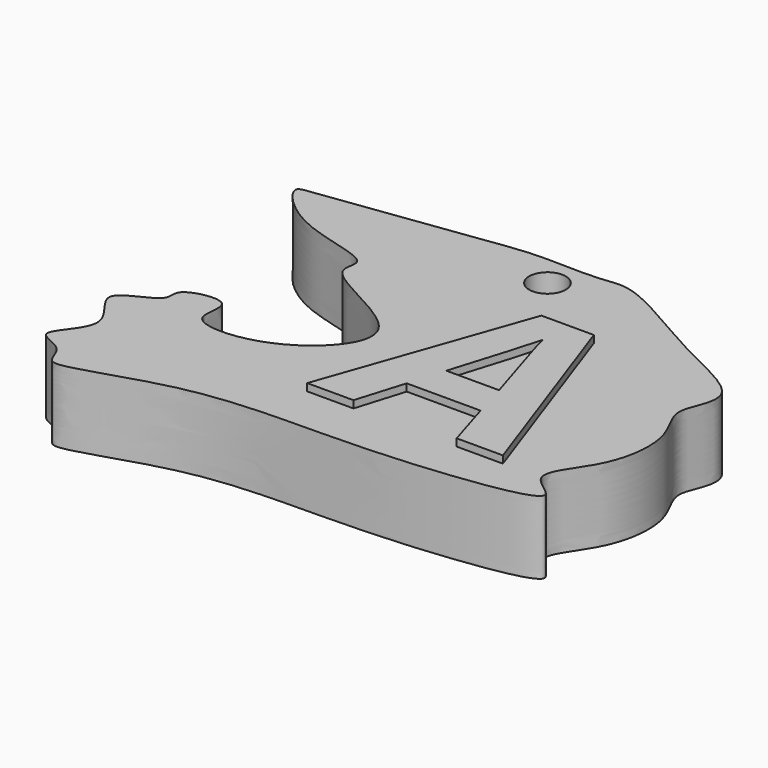
from build123d import *

# Parameters (mm, degrees)
F1_DEPTH     = 10
F2_TEXT_SIZE = 38.8719503664
F3_DEPTH     = 1
F5_D         = 5


# Not quite as in the source:
# - Text() gives the source's letters only with a copy of the font that has no kerning and outlines rounded to 1/6400 em; it was checked with that copy


with BuildPart() as f1:
    # F0 (on Top) → F1 (new body)
    with BuildSketch(Plane.XY):
        with BuildLine():
            add(Edge.make_bspline(
                [(-64.71713292, 51.556880079), (-62.588218655, 51.8064642414), (-54.5923947778, 52.9452082504), (-42.8082906348, 54.4694674172), (-36.54422944, 55.4457616296), (-28.0628023597, 54.8604905032), (-23.6071907873, 56.2361288313), (-11.7612832999, 48.5936441209), (-4.1799815494, 45.3962070939), (-0.4613117813, 42.5097622921), (-1.064368556, 39.231742487), (-2.8508041663, 35.8033968438), (1.0588645249, 31.1016218737), (0.1291140085, 21.6916004401), (-6.4423138044, 15.2417197866), (2.3773918907, 11.6389914958), (-14.074909308, 9.0603488589), (-29.0219761766, 8.4696762862), (-46.0852185761, 8.6454293617), (-59.7566922689, 3.1529002931), (-62.3297147196, 3.588226522), (-62.7184982721, 6.9655340487), (-68.4749409776, 7.8555551624), (-60.7053390885, 13.7573924), (-69.434806753, 19.8215393445), (-60.3239056166, 21.911121728), (-62.2881701416, 25.2528184799), (-54.4025753252, 26.8842302627), (-56.4195942983, 21.6120322246), (-53.1570896421, 19.8158876953), (-43.8341594361, 21.0472296338), (-33.803067045, 32.4464067053), (-52.7781031406, 38.01641813), (-48.7808171263, 43.2437903699), (-61.1954217995, 44.2443189742), (-67.4438826191, 51.2865017412), (-65.5770618435, 51.4560659488), (-64.71713292, 51.556880079)],
                knots=[0, 0, 0, 0, 0.034889454, 0.0736567381, 0.1021910124, 0.1334208485, 0.1569270481, 0.1976158714, 0.2307244074, 0.2526891338, 0.2715893387, 0.2920087933, 0.3176455683, 0.3515413752, 0.3811610008, 0.4034608881, 0.440394441, 0.4864913947, 0.5331707861, 0.5744962622, 0.5892703324, 0.6079898599, 0.6284399554, 0.655451093, 0.6830699922, 0.7093537072, 0.7260555182, 0.7509805891, 0.771683077, 0.7899033441, 0.8241097737, 0.8590954489, 0.9006324088, 0.9191202201, 0.9553579633, 0.9859071588, 1, 1, 1, 1], degree=3))
        make_face()
    extrude(amount=F1_DEPTH)

    # F2 (on face) → F3 (join)
    with BuildSketch(Plane.XY.offset(10)):
        with Locations((-36.0823199153, 15.2258016169)):
            Text('A', F2_TEXT_SIZE, font='Open Sans', font_style=FontStyle.BOLD, text_align=(TextAlign.LEFT, TextAlign.BOTTOM))
    extrude(amount=F3_DEPTH)

    # F5 (through all)
    with Locations(Plane.XY.offset(10)):
        with Locations((-31.6920727491, 50.8965365589)):
            Hole(F5_D / 2)


solid = f1.part
